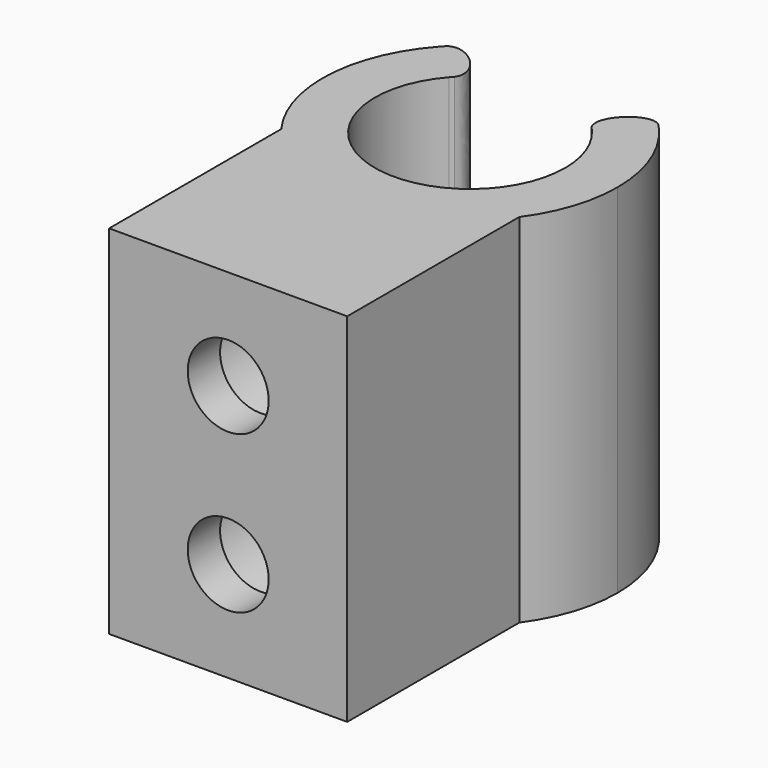
from build123d import *

# Parameters (mm, degrees)
F1_DEPTH = 15
F2_R     = 1.7
F3_DEPTH = 25
F2_R_2   = 2.9
F4_DEPTH = 11


# Not quite as in the source:
# - a feature names something its author has since deleted; it is built from what else it names


with BuildPart() as f1:
    # F0 (on Top) → F1 (new body)
    with BuildSketch(Plane.XY):
        with BuildLine():
            ThreePointArc((3, 2.6457513111), (3.7416573868, 1.4142135624), (4, 0))
            ThreePointArc((4, 0), (-1.4142135624, -3.7416573868), (-3, 2.6457513111))
            ThreePointArc((-3, 2.6457513111), (-2.9417354436, 2.7103860574), (-2.8820786357, 2.7737380442))
            add(Edge.make_bspline(
                [(-2.8820786357, 2.7737380442), (-2.3761359585, 3.4936148761), (-3.7454309361, 4.7943850499), (-4.4301631449, 4.3374709808)],
                knots=[0.118365038, 0.118365038, 0.118365038, 0.118365038, 2.0060809504, 2.0060809504, 2.0060809504, 2.0060809504], degree=3))
            ThreePointArc((-4.4301631449, 4.3374709808), (-4.524697766, 4.2387628061), (-4.6170335889, 4.1379947848))
            ThreePointArc((-4.6170335889, 4.1379947848), (-6.1925482399, 0.3038853354), (-5, -3.666060556))
            ThreePointArc((-5, -3.666060556), (0, -6.2), (5, -3.666060556))
            ThreePointArc((5, -3.666060556), (5.8923679451, -1.9287301522), (6.2, 0))
            ThreePointArc((6.2, 0), (5.7907516028, 2.2152191481), (4.6170335889, 4.1379947848))
            ThreePointArc((4.6170335889, 4.1379947848), (4.524697766, 4.2387628061), (4.4301631449, 4.3374709808))
            add(Edge.make_bspline(
                [(2.8820786357, 2.7737380442), (2.3761359585, 3.4936148761), (3.7454309361, 4.7943850499), (4.4301631449, 4.3374709808)],
                knots=[0.118365038, 0.118365038, 0.118365038, 0.118365038, 2.0060809504, 2.0060809504, 2.0060809504, 2.0060809504], degree=3))
            ThreePointArc((2.8820786357, 2.7737380442), (2.9417354436, 2.7103860574), (3, 2.6457513111))
        make_face()
        with BuildLine():
            ThreePointArc((5, -3.666060556), (0, -6.2), (-5, -3.666060556))
            Line((-5, -3.666060556), (-5, -12.7))
            Line((-5, -12.7), (0, -12.7))
            Line((0, -12.7), (5, -12.7))
            Line((5, -12.7), (5, -3.666060556))
        make_face()
    extrude(amount=F1_DEPTH)

    # F2 (on Front) → F3 (cut)
    with BuildSketch(Plane.XZ):
        with Locations((0, 10.8)):
            Circle(F2_R)
        with Locations((3.5e-09, 4.2)):
            Circle(F2_R)
    extrude(amount=F3_DEPTH, mode=Mode.SUBTRACT)

    # F2 (on Front) → F4 (cut)
    with BuildSketch(Plane.XZ):
        with Locations((0, 10.8)):
            Circle(F2_R_2)
        with Locations((0, 10.8)):
            Circle(F2_R, mode=Mode.SUBTRACT)
        with Locations((3.5e-09, 4.2)):
            Circle(F2_R_2)
        with Locations((3.5e-09, 4.2)):
            Circle(F2_R, mode=Mode.SUBTRACT)
    extrude(amount=F4_DEPTH, mode=Mode.SUBTRACT)


solid = f1.part
